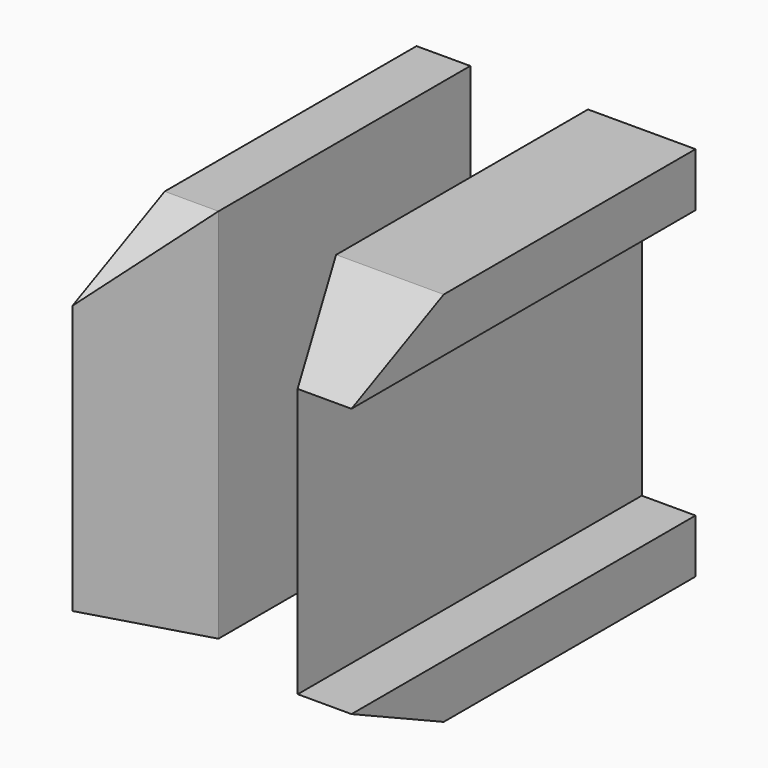
from build123d import *

# Parameters (mm, degrees)
F1_DEPTH = 50.8
F2_W     = 6.35
F2_H     = 44.45
F3_DEPTH = 50.8
F4_SIZE2 = 6.3366547667
F4_SIZE  = 13.589
F5_SIZE2 = 13.6176189452
F5_SIZE  = 6.35
F6_SIZE2 = 13.6176189452
F6_SIZE  = 6.35
F7_SIZE2 = 13.617609
F7_SIZE  = 6.34999


# Not quite as in the source:
# - a fillet or chamfer is up to 0.001 mm smaller than in the source, because OpenCascade refuses the exact size


with BuildPart() as f1:
    # F0 (on Front) → F1 (new body)
    with BuildSketch(Plane.XZ):
        Polygon((19.6477800332, 38.1), (19.6477800332, 44.45), (6.9477800332, 44.45), (6.9477800332, 0), (19.6477800332, 0), (19.6477800332, 6.35), (13.2977800332, 6.35), (13.2977800332, 38.1), align=None)
    extrude(amount=F1_DEPTH)

    # F4
    f4_edges = [f1.edges().sort_by_distance(p)[0] for p in [
        (6.94778, -50.8, 22.225),
    ]]
    f4_side = f1.faces().sort_by_distance((6.94778, -25.4, 22.225))[0]
    chamfer(f4_edges, length=F4_SIZE, length2=F4_SIZE2, reference=f4_side)

    # F5
    f5_edges = [f1.edges().sort_by_distance(p)[0] for p in [
        (16.466107, -50.8, 0),
    ]]
    f5_side = f1.faces().sort_by_distance((16.466107, -50.8, 44.000968))[0]
    chamfer(f5_edges, length=F5_SIZE, length2=F5_SIZE2, reference=f5_side)

    # F6
    f6_edges = [f1.edges().sort_by_distance(p)[0] for p in [
        (16.466107, -50.8, 44.45),
    ]]
    f6_side = f1.faces().sort_by_distance((16.43316, -50.8, 41.077314))[0]
    chamfer(f6_edges, length=F6_SIZE, length2=F6_SIZE2, reference=f6_side)


with BuildPart() as f3:
    # F2 (on Front) → F3 (new body)
    with BuildSketch(Plane.XZ):
        with Locations((-10.1346, 22.225)):
            Rectangle(F2_W, F2_H)
    extrude(amount=F3_DEPTH)

    # F7 (size 6.35 and 13.6176189452 in the source; OpenCascade refuses exactly that, so slightly less here)
    f7_edges = [f3.edges().sort_by_distance(p)[0] for p in [
        (-6.9596, -50.8, 22.225),
        (-10.1346, -50.8, 44.45),
        (-10.1346, -50.8, 0),
    ]]
    f7_side = f3.faces().sort_by_distance((-10.1346, -50.8, 22.225))[0]
    chamfer(f7_edges, length=F7_SIZE, length2=F7_SIZE2, reference=f7_side)


solid = Compound([f1.part, f3.part])
